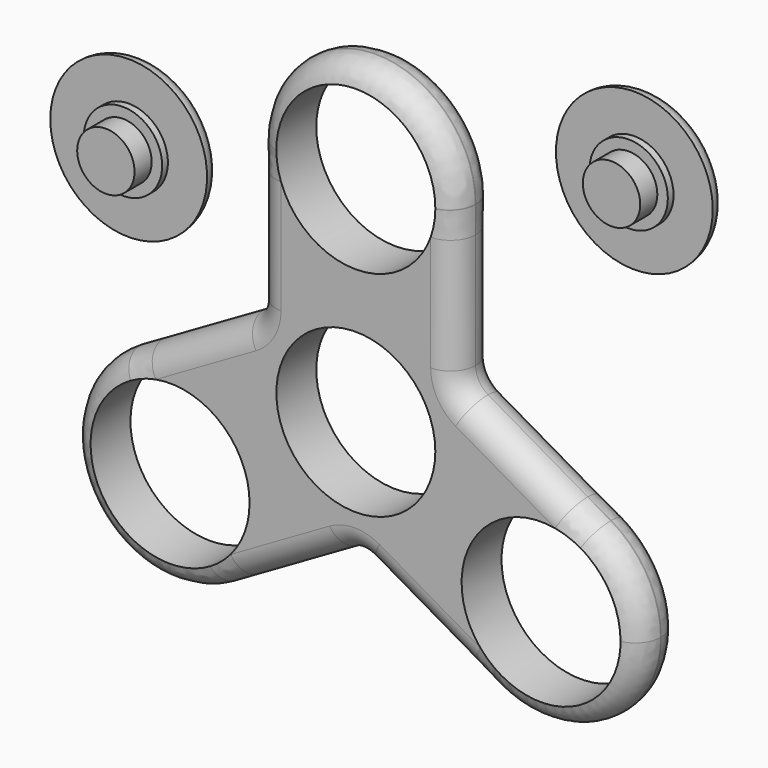
from build123d import *

# Parameters (mm, degrees)
F0_R     = 11.15
F1_DEPTH = 7
F2_R     = 11
F2_R_2   = 5.5
F3_DEPTH = 2.5
F2_R_3   = 4.025
F4_DEPTH = 3.5
F5_DEPTH = 6.5
F6_R     = 3.49999
F7_R     = 2.49999
F8_COUNT = 2


# Not quite as in the source:
# - a fillet or chamfer is up to 0.001 mm smaller than in the source, because OpenCascade refuses the exact size


with BuildPart() as f1:
    # F0 (on Front) → F1 (new body)
    with BuildSketch(Plane.XZ):
        with BuildLine():
            Line((-14, 15), (-14, -6.7050106472))
            Line((-14, -6.7050106472), (-33.0630497308, -17.7110675409))
            ThreePointArc((-33.0630497308, -17.7110675409), (-38.1874053838, -36.8354231939), (-19.0630497308, -41.9597788469))
            Line((-19.0630497308, -41.9597788469), (-0.1836715036, -31.0597647453))
            Line((-0.1836715036, -31.0597647453), (18.9807621135, -42.124355653))
            ThreePointArc((18.9807621135, -42.124355653), (38.1051177665, -37), (32.9807621135, -17.875644347))
            Line((32.9807621135, -17.875644347), (14, -6.9170962313))
            Line((14, -6.9170962313), (14, 15))
            ThreePointArc((14, 15), (0, 29), (-14, 15))
        make_face()
        with Locations((-26.0630497308, -29.8354231939)):
            Circle(F0_R, mode=Mode.SUBTRACT)
        with Locations((25.9807621135, -30)):
            Circle(F0_R, mode=Mode.SUBTRACT)
        with Locations((0, -15)):
            Circle(F0_R, mode=Mode.SUBTRACT)
        with Locations((0, 15)):
            Circle(F0_R, mode=Mode.SUBTRACT)
    extrude(amount=F1_DEPTH)

    # F6 (radius 3.5 in the source; OpenCascade refuses exactly that, so slightly less here)
    f6_edges = [f1.edges().sort_by_distance(p)[0] for p in [
        (-14, -3.5, 15),
        (-14, -3.5, -6.705011),
        (-14, 0, 4.147495),
        (-14, -7, 4.147495),
        (-33.06305, -3.5, -17.711068),
        (-23.531525, 0, -12.208039),
        (-23.531525, -7, -12.208039),
        (-19.06305, -3.5, -41.959779),
        (-38.187405, 0, -36.835423),
        (-38.187405, -7, -36.835423),
        (14, -3.5, 15),
        (0, 0, 29),
        (0, -7, 29),
        (-0.183672, -3.5, -31.059765),
        (-9.623361, 0, -36.509772),
        (-9.623361, -7, -36.509772),
        (18.980762, -3.5, -42.124356),
        (32.980762, -3.5, -17.875644),
        (38.105118, 0, -37),
        (38.105118, -7, -37),
        (9.398545, 0, -36.59206),
        (9.398545, -7, -36.59206),
        (14, -3.5, -6.917096),
        (23.490381, 0, -12.39637),
        (23.490381, -7, -12.39637),
        (14, 0, 4.041452),
        (14, -7, 4.041452),
    ]]
    fillet(f6_edges, radius=F6_R)


with BuildPart() as f3:
    # F2 (on Front) → F3 (new body)
    with BuildSketch(Plane.XZ):
        with Locations((35.4663021863, 24.5219450444)):
            Circle(F2_R)
        with Locations((35.4663021863, 24.5219450444)):
            Circle(F2_R_2, mode=Mode.SUBTRACT)
    extrude(amount=F3_DEPTH)

    # F2 (on Front) → F4 (join)
    with BuildSketch(Plane.XZ):
        with Locations((35.4663021863, 24.5219450444)):
            Circle(F2_R_2)
        with Locations((35.4663021863, 24.5219450444)):
            Circle(F2_R_3, mode=Mode.SUBTRACT)
    extrude(amount=F4_DEPTH)

    # F2 (on Front) → F5 (join)
    with BuildSketch(Plane.XZ):
        with Locations((35.4663021863, 24.5219450444)):
            Circle(F2_R_3)
    extrude(amount=F5_DEPTH)

    # F7 (radius 2.5 in the source; OpenCascade refuses exactly that, so slightly less here)
    f7_edges = [f3.edges().sort_by_distance(p)[0] for p in [
        (24.466302, 0, 24.521945),
    ]]
    fillet(f7_edges, radius=F7_R)


with BuildPart() as f8_1:
    # F8: instance of F3
    add(f3.part.rotate(Axis((0, 0, 15), (0, -1, 0)), 1 * 360 / F8_COUNT))


solid = Compound([f1.part, f3.part, f8_1.part])
